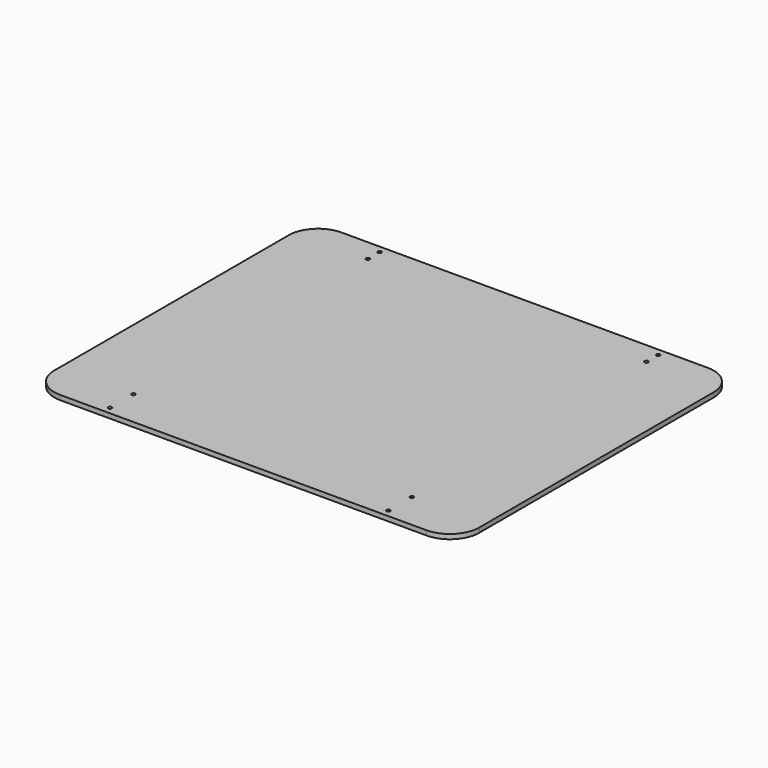
from build123d import *

# Parameters (mm, degrees)
F0_R     = 2.5
F1_DEPTH = 6.35


# Not quite as in the source:
# - a length typed as a fraction of an inch, garbled in the dataset ("3 / 203.2 mm" for 3/8 in), is restored


with BuildPart() as f1:
    # F0 (on Top) → F1 (new body)
    with BuildSketch(Plane.XY):
        with BuildLine():
            Line((-250, -240), (250, -240))
            ThreePointArc((250, -240), (278.2842712475, -228.2842712475), (290, -200))
            Line((290, -200), (290, 200))
            ThreePointArc((290, 200), (278.2842712475, 228.2842712475), (250, 240))
            Line((250, 240), (-250, 240))
            ThreePointArc((-250, 240), (-278.2842712475, 228.2842712475), (-290, 200))
            Line((-290, 200), (-290, -200))
            ThreePointArc((-290, -200), (-278.2842712475, -228.2842712475), (-250, -240))
        make_face()
        with Locations((-190, -230)):
            Circle(F0_R, mode=Mode.SUBTRACT)
        with Locations((-190, -190)):
            Circle(F0_R, mode=Mode.SUBTRACT)
        with Locations((190, -230)):
            Circle(F0_R, mode=Mode.SUBTRACT)
        with Locations((190, -190)):
            Circle(F0_R, mode=Mode.SUBTRACT)
        with Locations((-190, 210)):
            Circle(F0_R, mode=Mode.SUBTRACT)
        with Locations((-190, 230)):
            Circle(F0_R, mode=Mode.SUBTRACT)
        with BuildLine():
            ThreePointArc((190, 212.5), (191.767766953, 211.767766953), (192.5, 210))
            ThreePointArc((192.5, 210), (188.232233047, 208.232233047), (190, 212.5))
        make_face(mode=Mode.SUBTRACT)
        with BuildLine():
            ThreePointArc((192.5, 230), (191.767766953, 228.232233047), (190, 227.5))
            ThreePointArc((190, 227.5), (188.232233047, 231.767766953), (192.5, 230))
        make_face(mode=Mode.SUBTRACT)
    extrude(amount=-F1_DEPTH)


solid = f1.part
